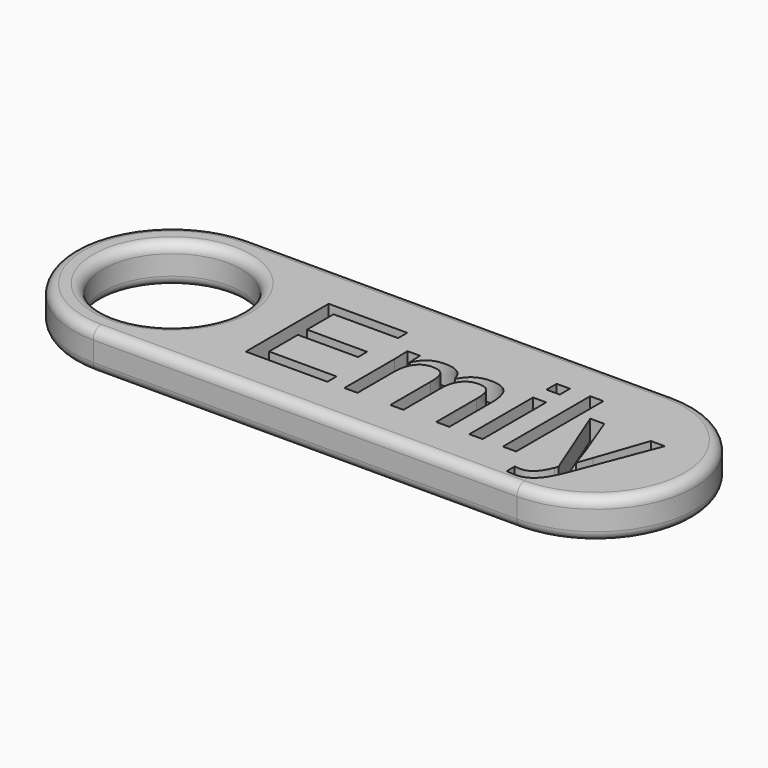
from build123d import *

# Parameters (mm, degrees)
F0_R         = 8.89
F1_DEPTH     = 5.08
F2_TEXT_SIZE = 19.4027777778
F3_DEPTH     = 2.54
F4_R         = 1.27


# Not quite as in the source:
# - Text() gives the source's letters only with a copy of the font that has no kerning and outlines rounded to 1/6400 em; it was checked with that copy


with BuildPart() as f1:
    # F0 (on Top) → F1 (new body)
    with BuildSketch(Plane.XY):
        with BuildLine():
            Line((-27.305, -12.7), (27.305, -12.7))
            ThreePointArc((27.305, -12.7), (40.005, 0), (27.305, 12.7))
            Line((27.305, 12.7), (-27.305, 12.7))
            ThreePointArc((-27.305, 12.7), (-40.005, 0), (-27.305, -12.7))
        make_face()
        with Locations((-27.305, 0)):
            Circle(F0_R, mode=Mode.SUBTRACT)
    extrude(amount=F1_DEPTH)

    # F2 (on face) → F3 (cut)
    with BuildSketch(Plane.XY.offset(5.08)):
        with Locations((-13.8123524306, -6.985)):
            Text('Emily', F2_TEXT_SIZE, font='Arimo', text_align=(TextAlign.LEFT, TextAlign.BOTTOM))
    extrude(amount=-F3_DEPTH, mode=Mode.SUBTRACT)

    # F4
    f4_edges = [f1.edges().sort_by_distance(p)[0] for p in [
        (-40.005, 0, 5.08),
        (0, -12.7, 0),
        (40.005, 0, 0),
        (0, 12.7, 0),
        (-40.005, 0, 0),
        (-36.195, 0, 0),
        (-36.195, 0, 5.08),
    ]]
    fillet(f4_edges, radius=F4_R)


solid = f1.part
